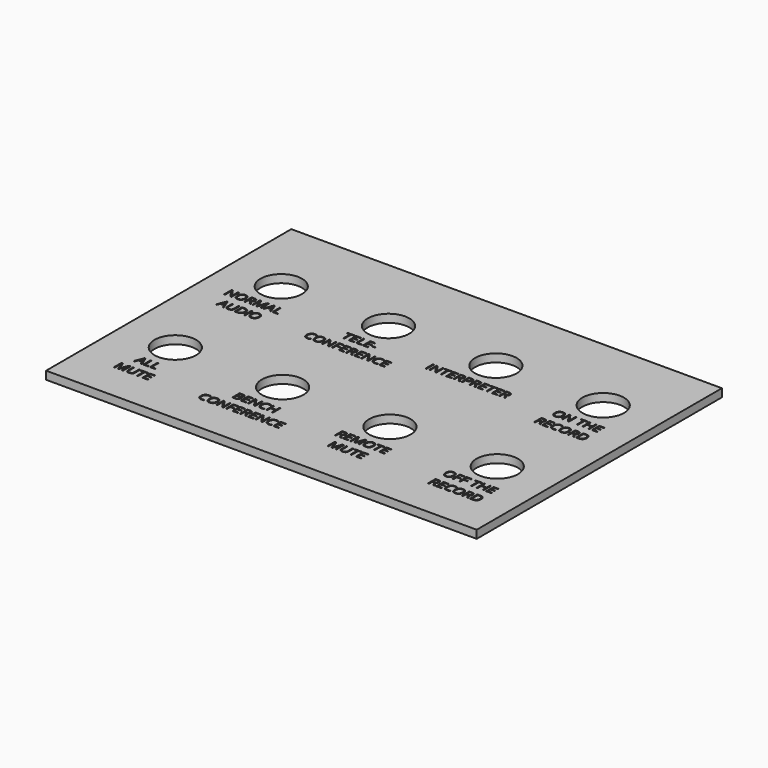
from build123d import *

# Parameters (mm, degrees)
F0_W         = 160.5
F0_H         = 114.25
F1_DEPTH     = 3
F2_R         = 7.75
F3_DEPTH     = 3
F4_TEXT_SIZE = 4.8611111111
F5_DEPTH     = 0.5


# Not quite as in the source:
# - Text() gives the source's letters only with a copy of the font that has no kerning and outlines rounded to 1/6400 em; it was checked with that copy


with BuildPart() as f1:
    # F0 (on Top) → F1 (new body)
    with BuildSketch(Plane.XY):
        Rectangle(F0_W, F0_H)
    extrude(amount=F1_DEPTH)

    # F2 (on face) → F3 (cut, through all)
    with BuildSketch(Plane.XY.offset(3)):
        with Locations((-60, 27.125)):
            Circle(F2_R)
        with Locations((-20, 27.125)):
            Circle(F2_R)
        with Locations((20, 27.125)):
            Circle(F2_R)
        with Locations((60, 27.125)):
            Circle(F2_R)
        with Locations((-60, -22.2286483815)):
            Circle(F2_R)
        with Locations((-20, -22.2286483815)):
            Circle(F2_R)
        with Locations((20, -22.2286483815)):
            Circle(F2_R)
        with Locations((60, -22.2286483815)):
            Circle(F2_R)
    extrude(amount=-F3_DEPTH, mode=Mode.SUBTRACT)

    # F4 (on face) → F5 (cut)
    with BuildSketch(Plane.XY.offset(3)):
        with Locations((-70.3234049479, 12.875)):
            Text('NORMAL', F4_TEXT_SIZE, font='Open Sans', text_align=(TextAlign.LEFT, TextAlign.BOTTOM))
        with Locations((-67.7971462674, 6.2638888889)):
            Text('AUDIO', F4_TEXT_SIZE, font='Open Sans', text_align=(TextAlign.LEFT, TextAlign.BOTTOM))
        with Locations((-26.6061740451, 12.875)):
            Text('TELE-', F4_TEXT_SIZE, font='Open Sans', text_align=(TextAlign.LEFT, TextAlign.BOTTOM))
        with Locations((-35.4480794271, 6.2638888889)):
            Text('CONFERENCE', F4_TEXT_SIZE, font='Open Sans', text_align=(TextAlign.LEFT, TextAlign.BOTTOM))
        with Locations((4.6590169271, 12.875)):
            Text('INTERPRETER', F4_TEXT_SIZE, font='Open Sans', text_align=(TextAlign.LEFT, TextAlign.BOTTOM))
        with Locations((51.6992730035, 12.875)):
            Text('ON THE', F4_TEXT_SIZE, font='Open Sans', text_align=(TextAlign.LEFT, TextAlign.BOTTOM))
        with Locations((50.4361436632, 6.2638888889)):
            Text('RECORD', F4_TEXT_SIZE, font='Open Sans', text_align=(TextAlign.LEFT, TextAlign.BOTTOM))
        with Locations((-64.1456163194, -36.4786483815)):
            Text('ALL', F4_TEXT_SIZE, font='Open Sans', text_align=(TextAlign.LEFT, TextAlign.BOTTOM))
        with Locations((-66.671875, -43.0897594926)):
            Text('MUTE', F4_TEXT_SIZE, font='Open Sans', text_align=(TextAlign.LEFT, TextAlign.BOTTOM))
        with Locations((-27.8693033854, -36.4786483815)):
            Text('BENCH', F4_TEXT_SIZE, font='Open Sans', text_align=(TextAlign.LEFT, TextAlign.BOTTOM))
        with Locations((-35.4480794271, -43.0897594926)):
            Text('CONFERENCE', F4_TEXT_SIZE, font='Open Sans', text_align=(TextAlign.LEFT, TextAlign.BOTTOM))
        with Locations((10.3506944444, -36.4786483815)):
            Text('REMOTE', F4_TEXT_SIZE, font='Open Sans', text_align=(TextAlign.LEFT, TextAlign.BOTTOM))
        with Locations((12.876953125, -43.0897594926)):
            Text('MUTE', F4_TEXT_SIZE, font='Open Sans', text_align=(TextAlign.LEFT, TextAlign.BOTTOM))
        with Locations((50.4361436632, -36.4786483815)):
            Text('OFF THE', F4_TEXT_SIZE, font='Open Sans', text_align=(TextAlign.LEFT, TextAlign.BOTTOM))
        with Locations((50.4361436632, -43.0897594926)):
            Text('RECORD', F4_TEXT_SIZE, font='Open Sans', text_align=(TextAlign.LEFT, TextAlign.BOTTOM))
    extrude(amount=-F5_DEPTH, mode=Mode.SUBTRACT)


solid = f1.part
